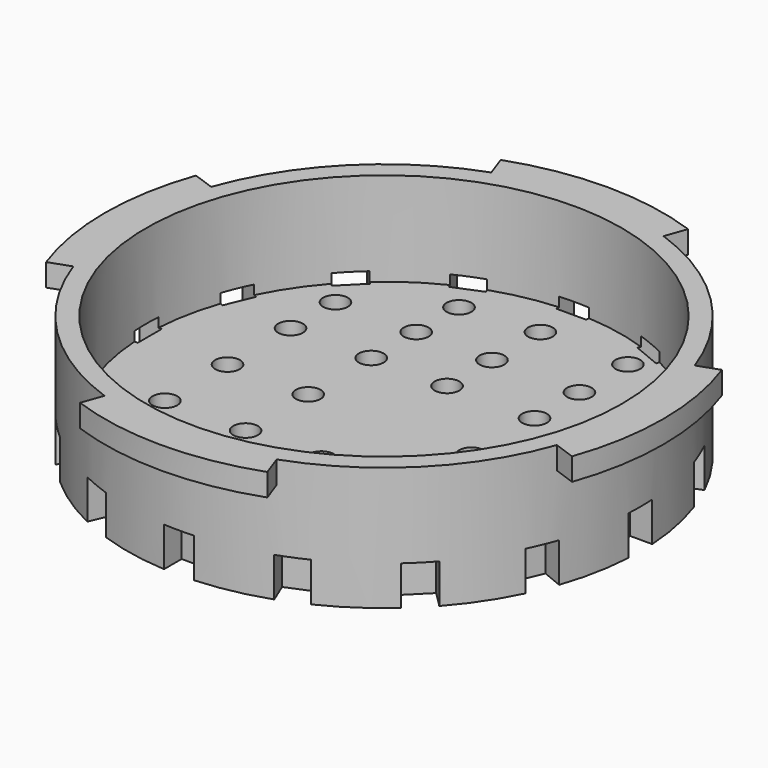
from build123d import *

# Parameters (mm, degrees)
F0_R     = 34.25
F0_R_2   = 31.75
F1_DEPTH = 16.5
F2_R     = 34.25
F2_R_2   = 31.75
F3_DEPTH = 4
F5_DEPTH = 5.25
F7_D     = 3.3
F9_DEPTH = 3


with BuildPart() as f1:
    # F0 (on Top) → F1 (new body)
    with BuildSketch(Plane.XY):
        Circle(F0_R)
        Circle(F0_R_2, mode=Mode.SUBTRACT)
    extrude(amount=F1_DEPTH)

    # F2 (on face) → F3 (join)
    with BuildSketch(Plane(origin=(0, 0, 0), x_dir=(1, 0, 0), z_dir=(0, 0, -1))):
        Circle(F2_R)
        Circle(F2_R_2, mode=Mode.SUBTRACT)
        Circle(F2_R_2)
    extrude(amount=-F3_DEPTH)

    # F4 (on face) → F5 (cut)
    with BuildSketch(Plane(origin=(0, 0, 0), x_dir=(1, 0, 0), z_dir=(0, 0, -1))):
        with BuildLine():
            ThreePointArc((25.5912946517, 22.762867527), (24.2184072556, 24.2184072556), (22.762867527, 25.5912946517))
            Line((22.762867527, 25.5912946517), (20.6828733497, 23.5113004745))
            Line((20.6828733497, 23.5113004745), (23.5113004745, 20.6828733497))
            Line((23.5113004745, 20.6828733497), (25.5912946517, 22.762867527))
        make_face()
        with BuildLine():
            ThreePointArc((14.9323010635, 30.8235118854), (13.1069075585, 31.6428739885), (11.2367829334, 32.3542456149))
            Line((11.2367829334, 32.3542456149), (10.1110981964, 29.6366022557))
            Line((10.1110981964, 29.6366022557), (13.8066163264, 28.1058685262))
            Line((13.8066163264, 28.1058685262), (14.9323010635, 30.8235118854))
        make_face()
        with BuildLine():
            ThreePointArc((2, 34.1915559751), (0, 34.25), (-2, 34.1915559751))
            Line((-2, 34.1915559751), (-2, 31.25))
            Line((-2, 31.25), (2, 31.25))
            Line((2, 31.25), (2, 34.1915559751))
        make_face()
        with BuildLine():
            Line((-10.1110981964, 29.6366022557), (-11.2367829334, 32.3542456149))
            ThreePointArc((-11.2367829334, 32.3542456149), (-13.1069075585, 31.6428739885), (-14.9323010635, 30.8235118854))
            Line((-14.9323010635, 30.8235118854), (-13.8066163264, 28.1058685262))
            Line((-13.8066163264, 28.1058685262), (-10.1110981964, 29.6366022557))
        make_face()
        with BuildLine():
            Line((-20.6828733497, 23.5113004745), (-22.762867527, 25.5912946517))
            ThreePointArc((-22.762867527, 25.5912946517), (-24.2184072556, 24.2184072556), (-25.5912946517, 22.762867527))
            Line((-25.5912946517, 22.762867527), (-23.5113004745, 20.6828733497))
            Line((-23.5113004745, 20.6828733497), (-20.6828733497, 23.5113004745))
        make_face()
        with BuildLine():
            Line((-31.25, 2), (-34.1915559751, 2))
            ThreePointArc((-34.1915559751, 2), (-34.25, 0), (-34.1915559751, -2))
            Line((-34.1915559751, -2), (-31.25, -2))
            Line((-31.25, -2), (-31.25, 2))
        make_face()
        with BuildLine():
            Line((-29.6366022557, -10.1110981964), (-32.3542456149, -11.2367829334))
            ThreePointArc((-32.3542456149, -11.2367829334), (-31.6428739885, -13.1069075585), (-30.8235118854, -14.9323010635))
            Line((-30.8235118854, -14.9323010635), (-28.1058685262, -13.8066163264))
            Line((-28.1058685262, -13.8066163264), (-29.6366022557, -10.1110981964))
        make_face()
        with BuildLine():
            Line((-23.5113004745, -20.6828733497), (-25.5912946517, -22.762867527))
            ThreePointArc((-25.5912946517, -22.762867527), (-24.2184072556, -24.2184072556), (-22.762867527, -25.5912946517))
            Line((-22.762867527, -25.5912946517), (-20.6828733497, -23.5113004745))
            Line((-20.6828733497, -23.5113004745), (-23.5113004745, -20.6828733497))
        make_face()
        with BuildLine():
            Line((-13.8066163264, -28.1058685262), (-14.9323010635, -30.8235118854))
            ThreePointArc((-14.9323010635, -30.8235118854), (-13.1069075585, -31.6428739885), (-11.2367829334, -32.3542456149))
            Line((-11.2367829334, -32.3542456149), (-10.1110981964, -29.6366022557))
            Line((-10.1110981964, -29.6366022557), (-13.8066163264, -28.1058685262))
        make_face()
        with BuildLine():
            Line((-2, -31.25), (-2, -34.1915559751))
            ThreePointArc((-2, -34.1915559751), (0, -34.25), (2, -34.1915559751))
            Line((2, -34.1915559751), (2, -31.25))
            Line((2, -31.25), (-2, -31.25))
        make_face()
        with BuildLine():
            ThreePointArc((11.2367829334, -32.3542456149), (13.1069075585, -31.6428739885), (14.9323010635, -30.8235118854))
            Line((14.9323010635, -30.8235118854), (13.8066163264, -28.1058685262))
            Line((13.8066163264, -28.1058685262), (10.1110981964, -29.6366022557))
            Line((10.1110981964, -29.6366022557), (11.2367829334, -32.3542456149))
        make_face()
        with BuildLine():
            ThreePointArc((30.8235118854, -14.9323010635), (31.6428739885, -13.1069075585), (32.3542456149, -11.2367829334))
            Line((32.3542456149, -11.2367829334), (29.6366022557, -10.1110981964))
            Line((29.6366022557, -10.1110981964), (28.1058685262, -13.8066163264))
            Line((28.1058685262, -13.8066163264), (30.8235118854, -14.9323010635))
        make_face()
        with BuildLine():
            ThreePointArc((22.762867527, -25.5912946517), (24.2184072556, -24.2184072556), (25.5912946517, -22.762867527))
            Line((25.5912946517, -22.762867527), (23.5113004745, -20.6828733497))
            Line((23.5113004745, -20.6828733497), (20.6828733497, -23.5113004745))
            Line((20.6828733497, -23.5113004745), (22.762867527, -25.5912946517))
        make_face()
        with BuildLine():
            ThreePointArc((34.25, 0), (34.2353858759, 1.0004268719), (34.1915559751, 2))
            Line((34.1915559751, 2), (31.25, 2))
            Line((31.25, 2), (31.25, -2))
            Line((31.25, -2), (34.1915559751, -2))
            ThreePointArc((34.1915559751, -2), (34.2353858759, -1.0004268719), (34.25, 0))
        make_face()
        with BuildLine():
            ThreePointArc((32.3542456149, 11.2367829334), (31.6428739885, 13.1069075585), (30.8235118854, 14.9323010635))
            Line((30.8235118854, 14.9323010635), (28.1058685262, 13.8066163264))
            Line((28.1058685262, 13.8066163264), (29.6366022557, 10.1110981964))
            Line((29.6366022557, 10.1110981964), (32.3542456149, 11.2367829334))
        make_face()
        with BuildLine():
            Line((-28.1058685262, 13.8066163264), (-30.8235118854, 14.9323010635))
            ThreePointArc((-30.8235118854, 14.9323010635), (-31.6428739885, 13.1069075585), (-32.3542456149, 11.2367829334))
            Line((-32.3542456149, 11.2367829334), (-29.6366022557, 10.1110981964))
            Line((-29.6366022557, 10.1110981964), (-28.1058685262, 13.8066163264))
        make_face()
    extrude(amount=-F5_DEPTH, mode=Mode.SUBTRACT)

    # F7 (through all)
    with Locations(Plane(origin=(0, 0, 0), x_dir=(1, 0, 0), z_dir=(0, 0, -1))):
        with Locations((-10.1110981964, 0), (-10.1110981964, 10.4496451095), (-10.1110981964, 17.7097469568), (-20.8794418722, 17.7097469568), (-20.8794418722, 10.4496451095), (-20.8794418722, 0), (-20.8794418722, -10.5109745637), (-20.8794418722, -18.0052742362), (-10.1110981964, -25.1482781023), (-10.1110981964, -18.0052742362), (-10.1110981964, -10.5109745637), (0, -18.0052742362), (0, -10.5109745637), (0, -26.0850638151), (0, 10.4496451095), (0, 17.7097469568), (-10.1110981964, 25.5912946517), (11.6739207879, 25.5912946517), (0, 25.906637311), (11.6739207879, 17.7097469568), (11.6739207879, 10.4496451095), (11.6739207879, 0), (11.6739207879, -10.5109745637), (11.6739207879, -26.0850638151), (21.3930904865, -18.0052742362), (11.6739207879, -18.0052742362), (21.3930904865, -10.5109745637), (21.3930904865, 0), (21.3930904865, 10.4496451095), (21.3930904865, 17.7097469568)):
            Hole(F7_D / 2)

    # F8 (on face) → F9 (join)
    with BuildSketch(Plane.XY.offset(16.5)):
        with BuildLine():
            ThreePointArc((-32.2640173781, -11.4932885906), (-34.25, 0), (-32.2640173781, 11.4932885906))
            Line((-32.2640173781, 11.4932885906), (-35.0900626959, 12.5))
            ThreePointArc((-35.0900626959, 12.5), (-37.25, 0), (-35.0900626959, -12.5))
            Line((-35.0900626959, -12.5), (-32.2640173781, -11.4932885906))
        make_face()
        with BuildLine():
            Line((11.4932885906, 32.2640173781), (12.5, 35.0900626959))
            ThreePointArc((12.5, 35.0900626959), (0, 37.25), (-12.5, 35.0900626959))
            Line((-12.5, 35.0900626959), (-11.4932885906, 32.2640173781))
            ThreePointArc((-11.4932885906, 32.2640173781), (0, 34.25), (11.4932885906, 32.2640173781))
        make_face()
        with BuildLine():
            Line((35.0900626959, 12.5), (32.2640173781, 11.4932885906))
            ThreePointArc((32.2640173781, 11.4932885906), (33.7498525567, 5.8318052437), (34.25, 0))
            ThreePointArc((34.25, 0), (33.7498525567, -5.8318052437), (32.2640173781, -11.4932885906))
            Line((32.2640173781, -11.4932885906), (35.0900626959, -12.5))
            ThreePointArc((35.0900626959, -12.5), (37.25, 0), (35.0900626959, 12.5))
        make_face()
        with BuildLine():
            ThreePointArc((11.4932885906, -32.2640173781), (0, -34.25), (-11.4932885906, -32.2640173781))
            Line((-11.4932885906, -32.2640173781), (-12.5, -35.0900626959))
            ThreePointArc((-12.5, -35.0900626959), (0, -37.25), (12.5, -35.0900626959))
            Line((12.5, -35.0900626959), (11.4932885906, -32.2640173781))
        make_face()
    extrude(amount=-F9_DEPTH)


solid = f1.part
